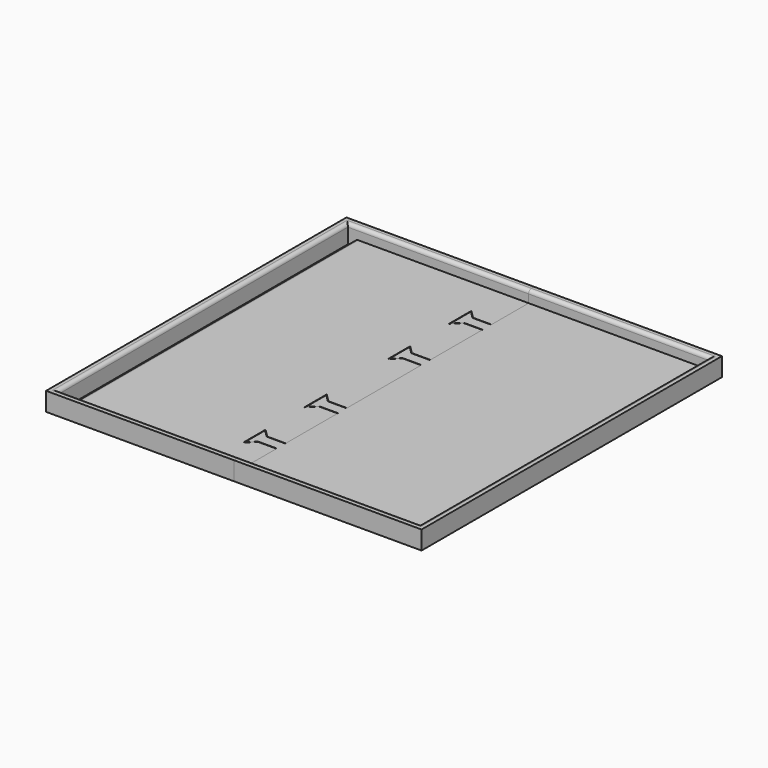
from build123d import *

# Parameters (mm, degrees)
F1_DEPTH = 8
F2_DEPTH = 3
F3_DEPTH = 3
F4_DEPTH = 8
F5_R     = 1.5
F5_2_R   = 1.5


with BuildPart() as f1:
    # F0 (on Top) → F1 (new body)
    with BuildSketch(Plane.XY):
        Polygon((-39, -39), (-39, 39), (-36, 39), (39, 39), (39, 42), (-42, 42), (-42, -39), (-42, -120), (39, -120), (39, -117), (-36, -117), (-39, -117), align=None)
    extrude(amount=F1_DEPTH)

    # F0 (on Top) → F2 (join)
    with BuildSketch(Plane.XY):
        Polygon((39, 39), (-36, 39), (-36, -117), (39, -117), (39, -97), (31, -97), (27.4644660941, -100.5355339059), (27.4644660941, -88.4644660941), (31, -92), (39, -92), (39, -64), (31, -64), (27.4644660941, -67.5355339059), (27.4644660941, -55.4644660941), (31, -59), (39, -59), (39, -19), (31, -19), (27.4644660941, -22.5355339059), (27.4644660941, -10.4644660941), (31, -14), (39, -14), (39, 14), (31, 14), (27.4644660941, 10.4644660941), (27.4644660941, 22.5355339059), (31, 19), (39, 19), align=None)
    extrude(amount=F2_DEPTH)

    # F5
    f5_edges = [f1.edges().sort_by_distance(p)[0] for p in [
        (0, 39, 8),
        (0, -117, 8),
        (-39, -39, 8),
        (-36, -39, 3),
    ]]
    fillet(f5_edges, radius=F5_R)


with BuildPart() as f3:
    # F0 (on Top) → F3 (new body)
    with BuildSketch(Plane.XY):
        Polygon((114, 39), (39, 39), (39, 19), (39, 18.8), (39, 14.2), (39, 14), (39, -14), (39, -14.2), (39, -18.8), (39, -19), (39, -59), (39, -59.2), (39, -63.8), (39, -64), (39, -92), (39, -92.2), (39, -96.8), (39, -97), (39, -117), (114, -117), align=None)
        Polygon((39, 42), (39, 39), (114, 39), (117, 39), (117, -39), (117, -117), (114, -117), (39, -117), (39, -120), (120, -120), (120, -39), (120, 42), align=None)
        Polygon((30.9171572875, -96.8), (39, -96.8), (39, -92.2), (30.9171572875, -92.2), (27.6644660941, -88.9473088065), (27.6644660941, -100.0526911935), align=None)
        Polygon((30.9171572875, -63.8), (39, -63.8), (39, -59.2), (30.9171572875, -59.2), (27.6644660941, -55.9473088065), (27.6644660941, -67.0526911935), align=None)
        Polygon((39, -18.8), (39, -14.2), (30.9171572875, -14.2), (27.6644660941, -10.9473088065), (27.6644660941, -22.0526911935), (30.9171572875, -18.8), align=None)
        Polygon((39, 14.2), (39, 18.8), (30.9171572875, 18.8), (27.6644660941, 22.0526911935), (27.6644660941, 10.9473088065), (30.9171572875, 14.2), align=None)
    extrude(amount=F3_DEPTH)

    # F0 (on Top) → F4 (join)
    with BuildSketch(Plane.XY):
        Polygon((39, 42), (39, 39), (114, 39), (117, 39), (117, -39), (117, -117), (114, -117), (39, -117), (39, -120), (120, -120), (120, -39), (120, 42), align=None)
    extrude(amount=F4_DEPTH)

    # F5#2
    f5_2_edges = [f3.edges().sort_by_distance(p)[0] for p in [
        (78, 39, 8),
        (117, -39, 8),
        (78, -117, 8),
        (114, -39, 3),
    ]]
    fillet(f5_2_edges, radius=F5_2_R)


solid = Compound([f1.part, f3.part])
